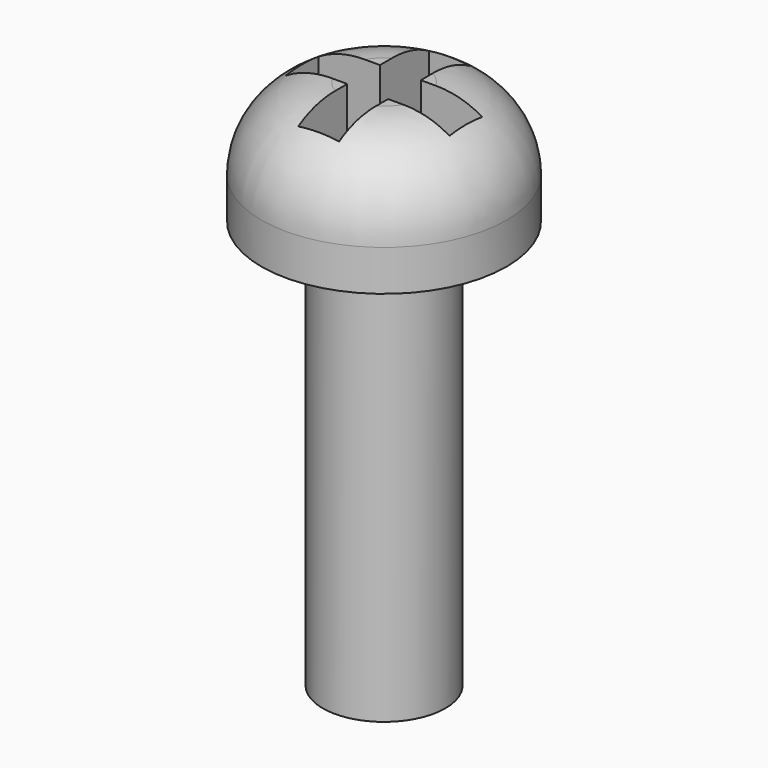
from build123d import *

# Parameters (mm, degrees)
F0_R     = 1.5
F1_DEPTH = 10
F2_R     = 3
F2_R_2   = 1.5
F3_DEPTH = 3
F4_W     = 1.5
F4_H     = 1
F4_W_2   = 1
F4_H_2   = 1.5
F5_DEPTH = 2


# Not quite as in the source:
# - a fillet or chamfer that OpenCascade refuses, or shapes differently, is made with other operations: its cross-section is extruded or revolved along the edge and cut away or added


with BuildPart() as f1:
    # F0 (on Top) → F1 (new body)
    with BuildSketch(Plane.XY):
        Circle(F0_R)
    extrude(amount=-F1_DEPTH)

    # F2 (on face) → F3 (join)
    with BuildSketch(Plane.XY):
        Circle(F2_R)
        Circle(F2_R_2, mode=Mode.SUBTRACT)
        Circle(F2_R_2)
    extrude(amount=F3_DEPTH)

    # F4 (on face) → F5 (cut)
    with BuildSketch(Plane.XY.offset(3)):
        with Locations((-1.25, 0)):
            Rectangle(F4_W, F4_H)
        with Locations((0, 1.25)):
            Rectangle(F4_W_2, F4_H_2)
        Rectangle(F4_W_2, F4_H)
        with Locations((1.25, 0)):
            Rectangle(F4_W, F4_H)
        with Locations((0, -1.25)):
            Rectangle(F4_W_2, F4_H_2)
    extrude(amount=-F5_DEPTH, mode=Mode.SUBTRACT)

    # F6: fillet of radius 2 on 1 edges, made by hand

    # F6_s1 → F6_t2 (revolve, cut)
    with BuildSketch(Plane.XZ):
        with BuildLine():
            ThreePointArc((3, 1), (2.4142135624, 2.4142135624), (1, 3))
            Line((1, 3), (3, 3))
            Line((3, 3), (3, 1))
        make_face()
    revolve(axis=Axis((0, 0, 3), (0, 0, 1)), mode=Mode.SUBTRACT)


solid = f1.part
